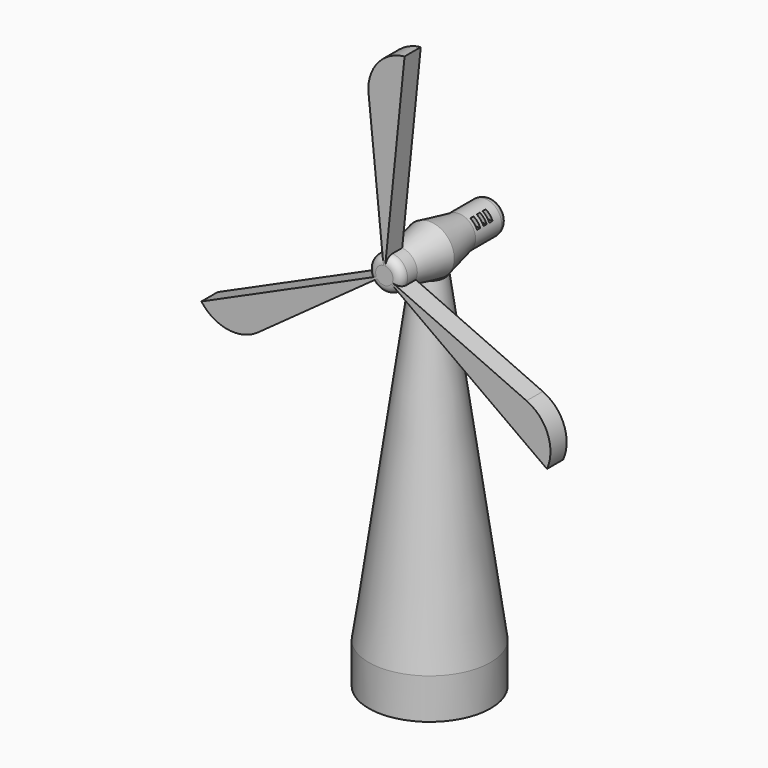
from build123d import *

# Parameters (mm, degrees)
F0_R          = 38.2277383981
F1_DEPTH      = 203.2
F1_TAPER      = 8
F1_DEPTH_BACK = 25.4
F2_R          = 15.390866947
F3_DEPTH      = 22.86
F3_TAPER      = 12
F4_R          = 10.5318239472
F5_DEPTH      = 6.35
F6_DEPTH      = 6.35
F7_R          = 5.08
F9_DEPTH      = 12.7
F10_T1_DEPTH  = 152.5201677194
F11_DEPTH     = 25.4
F12_R         = 5.08
F13_W         = 2.54
F13_H         = 5.08
F14_DEPTH     = 25.4


# Not quite as in the source:
# - a fillet or chamfer that OpenCascade refuses, or shapes differently, is made with other operations: its cross-section is extruded or revolved along the edge and cut away or added


with BuildPart() as f1:
    # F0 (on Top) → F1 (new body, two sides)
    with BuildSketch(Plane.XY) as f1_sk:
        Circle(F0_R)
    extrude(amount=F1_DEPTH, taper=F1_TAPER)
    extrude(f1_sk.sketch, amount=-F1_DEPTH_BACK)

    # F2 (on Front) → F3 (join, symmetric)
    with BuildSketch(Plane.XZ):
        with Locations((0, 215.6233489513)):
            Circle(F2_R)
    extrude(amount=F3_DEPTH, both=True, taper=F3_TAPER)

    # F4 (on face) → F5 (join)
    with BuildSketch(Plane.XZ.offset(22.86)):
        with Locations((0, 215.6233489513)):
            Circle(F4_R)
    extrude(amount=F5_DEPTH)

    # F6 (add): a face of the model
    f6_faces = [f1.faces().sort_by_distance(p)[0] for p in [
        (0, -29.21, 215.6233489513),
    ]]
    extrude(f6_faces, amount=F6_DEPTH)

    # F7
    f7_edges = [f1.edges().sort_by_distance(p)[0] for p in [
        (-10.531824, -35.56, 215.623349),
    ]]
    fillet(f7_edges, radius=F7_R)

    # F8 (on face) → F9 (join)
    with BuildSketch(Plane.XZ.offset(35.56)):
        with BuildLine():
            Line((12.7, 340.7739359743), (0, 340.7739359743))
            Line((0, 340.7739359743), (-12.7, 340.7739359743))
            Line((-12.7, 340.7739359743), (-0.5504120884, 221.0473171375))
            ThreePointArc((-0.5504120884, 221.0473171375), (0, 221.0751728985), (0.5504120884, 221.0473171375))
            Line((0.5504120884, 221.0473171375), (12.7, 340.7739359743))
        make_face()
        with BuildLine():
            ThreePointArc((-4.4220881943, 212.4346940072), (-4.7214180352, 212.8974369777), (-4.9725002827, 213.3880357094))
            Line((-4.9725002827, 213.3880357094), (-114.7335876604, 164.0465780679))
            Line((-114.7335876604, 164.0465780679), (-108.3835876604, 153.0480554399))
            Line((-108.3835876604, 153.0480554399), (-102.0335876604, 142.0495328118))
            Line((-102.0335876604, 142.0495328118), (-4.4220881943, 212.4346940072))
        make_face()
        with BuildLine():
            Line((114.7335876604, 164.0465780679), (4.9725002827, 213.3880357094))
            ThreePointArc((4.9725002827, 213.3880357094), (4.7214180352, 212.8974369777), (4.4220881943, 212.4346940072))
            Line((4.4220881943, 212.4346940072), (102.0335876604, 142.0495328118))
            Line((102.0335876604, 142.0495328118), (108.3835876604, 153.0480554399))
            Line((108.3835876604, 153.0480554399), (114.7335876604, 164.0465780679))
        make_face()
    extrude(amount=-F9_DEPTH)

    # F10: fillet of radius 25.4 on 3 edges, made by hand

    # F10_s2 → F10_t1 (cut)
    with BuildSketch(Plane.XZ.offset(-47.0500838597)):
        with BuildLine():
            ThreePointArc((-9.8767719847, 312.9527829497), (-4.3295288952, 331.5222775929), (12.7, 340.7739359743))
            Line((12.7, 340.7739359743), (-12.7, 340.7739359743))
            Line((-12.7, 340.7739359743), (-9.8767719847, 312.9527829497))
        make_face()
        with BuildLine():
            ThreePointArc((-79.3513763862, 158.405096506), (-98.2066520274, 153.9244026208), (-114.7335876604, 164.0465780679))
            Line((-114.7335876604, 164.0465780679), (-102.0335876604, 142.0495328118))
            Line((-102.0335876604, 142.0495328118), (-79.3513763862, 158.405096506))
        make_face()
        with BuildLine():
            ThreePointArc((89.2281483709, 175.5121673983), (102.5361809226, 161.4233666402), (102.0335876604, 142.0495328118))
            Line((102.0335876604, 142.0495328118), (114.7335876604, 164.0465780679))
            Line((114.7335876604, 164.0465780679), (89.2281483709, 175.5121673983))
        make_face()
    extrude(amount=F10_T1_DEPTH, mode=Mode.SUBTRACT)

    # F11 (add): a face of the model
    f11_faces = [f1.faces().sort_by_distance(p)[0] for p in [
        (0, 22.86, 215.6233489513),
    ]]
    extrude(f11_faces, amount=F11_DEPTH)

    # F12
    f12_edges = [f1.edges().sort_by_distance(p)[0] for p in [
        (-10.531824, 48.26, 215.623349),
    ]]
    fillet(f12_edges, radius=F12_R)

    # F13 (on Right) → F14 (cut)
    with BuildSketch(Plane.YZ):
        with Locations((31.1770738256, 222.0274733686)):
            Rectangle(F13_W, F13_H)
        with Locations((26.1536446553, 222.0274733686)):
            Rectangle(F13_W, F13_H)
        with Locations((35.7572549176, 222.0274733686)):
            Rectangle(F13_W, F13_H)
    extrude(amount=F14_DEPTH, mode=Mode.SUBTRACT)


solid = f1.part
